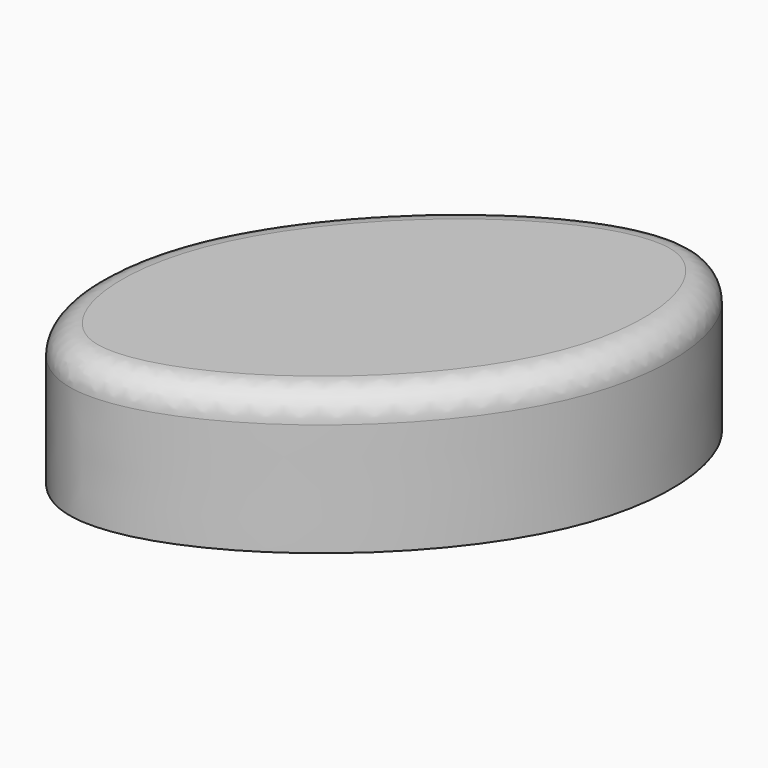
from build123d import *

# Parameters (mm, degrees)
F1_DEPTH = 25.4
F2_R     = 5.08


with BuildPart() as f1:
    # F0 (on Top) → F1 (new body)
    with BuildSketch(Plane.XY):
        with BuildLine():
            add(Edge.make_bspline(
                [(-57.8798130155, -40.8128574491), (-70.589949562, -37.2799462901), (-79.9950231197, 6.4510198683), (-3.0329710098, 63.8722881838), (14.0999933382, -6.9425561353), (-41.3351215167, -45.4116219865), (-57.8798130155, -40.8128574491)],
                knots=[0, 0, 0, 0, 0.2165900832, 0.4983404404, 0.7180662777, 1, 1, 1, 1], degree=3))
        make_face()
    extrude(amount=F1_DEPTH)

    # F2
    f2_edges = [f1.edges().sort_by_distance(p)[0] for p in [
        (-9.165176, 41.652267, 25.4),
    ]]
    fillet(f2_edges, radius=F2_R)


solid = f1.part
